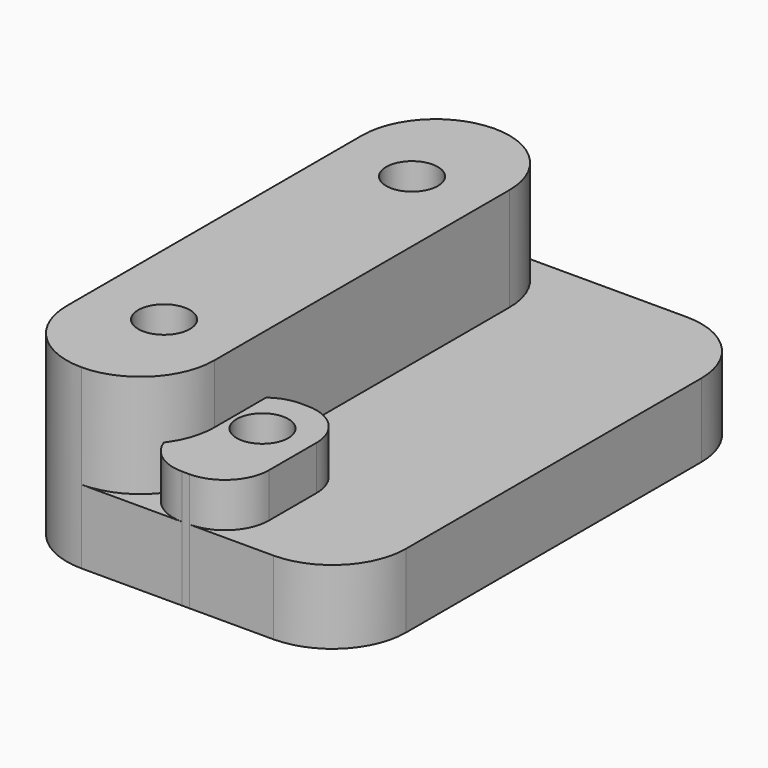
from build123d import *

# Parameters (mm, degrees)
F0_W     = 23
F0_H     = 35
F1_DEPTH = 5
F2_W     = 10
F2_H     = 35
F3_DEPTH = 7
F4_R     = 1.75
F5_DEPTH = 12
F6_R     = 4.99999
F7_W     = 6.5
F7_H     = 10
F7_R     = 1.75
F8_DEPTH = 8
F9_R     = 3


# Not quite as in the source:
# - a fillet or chamfer is up to 0.001 mm smaller than in the source, because OpenCascade refuses the exact size


with BuildPart() as f1:
    # F0 (on Top) → F1 (new body)
    with BuildSketch(Plane.XY):
        with Locations((2.6824958399, 17.5)):
            Rectangle(F0_W, F0_H)
    extrude(amount=F1_DEPTH)

    # F2 (on face) → F3 (join)
    with BuildSketch(Plane.XY.offset(5)):
        with Locations((-3.8175041601, 17.5)):
            Rectangle(F2_W, F2_H)
    extrude(amount=F3_DEPTH)

    # F4 (on face) → F5 (cut, through all)
    with BuildSketch(Plane.XY.offset(12)):
        with Locations((-3.8175041601, 28)):
            Circle(F4_R)
        with Locations((-3.8175041601, 7)):
            Circle(F4_R)
    extrude(amount=-F5_DEPTH, mode=Mode.SUBTRACT)

    # F6 (radius 5 in the source; OpenCascade refuses exactly that, so slightly less here)
    f6_edges = [f1.edges().sort_by_distance(p)[0] for p in [
        (-8.817504, 35, 6),
        (1.182496, 35, 8.5),
        (-8.817504, 0, 6),
        (1.182496, 0, 8.5),
        (14.182496, 0, 2.5),
        (14.182496, 35, 2.5),
    ]]
    fillet(f6_edges, radius=F6_R)


with BuildPart() as f8:
    # F7 (on Top) → F8 (new body)
    with BuildSketch(Plane.XY):
        with Locations((3.25, 5)):
            Rectangle(F7_W, F7_H)
        with Locations((3.25, 6.5)):
            Circle(F7_R, mode=Mode.SUBTRACT)
    extrude(amount=F8_DEPTH)

    # F9
    f9_edges = [f8.edges().sort_by_distance(p)[0] for p in [
        (6.5, 0, 4),
        (6.5, 10, 4),
        (0, 0, 4),
        (0, 10, 4),
    ]]
    fillet(f9_edges, radius=F9_R)


solid = Compound([f1.part, f8.part])
